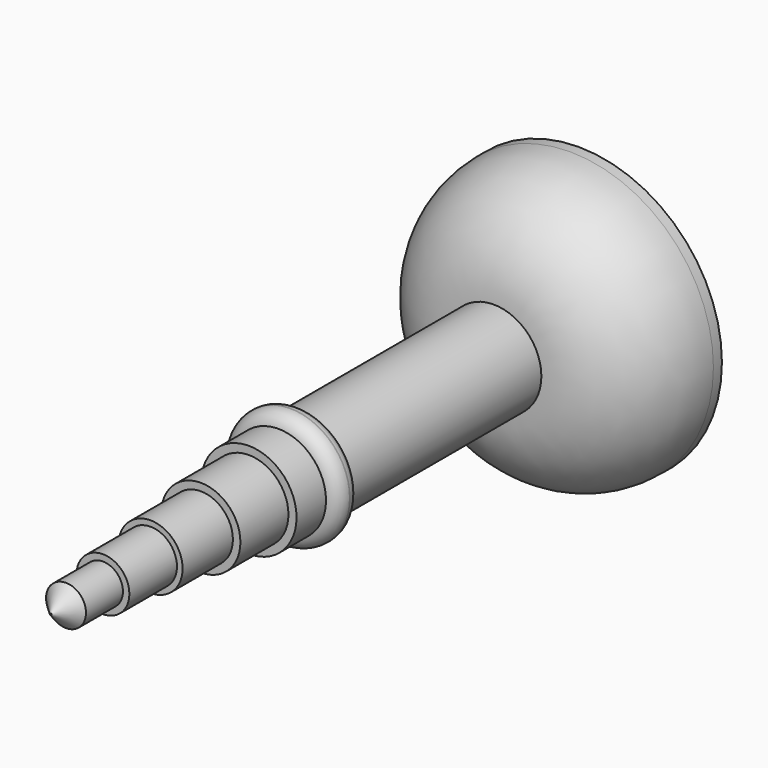
from build123d import *

# Parameters (mm, degrees)
F0_R      = 34.2582763281
F1_DEPTH  = 25.4
F2_R      = 22.86
F3_DEPTH  = 57.9221248627
F4_R      = 14.2196111498
F4_R_2    = 11.3982763281
F5_DEPTH  = 6.4626615494
F7_R      = 2.794
F8_DEPTH  = 15.2733121067
F9_R      = 9.4619725581
F10_DEPTH = 14.3653638661
F11_R     = 7.6680324081
F12_DEPTH = 15.0388088077
F13_R     = 6.3210744691
F14_DEPTH = 14.2291132361
F15_R     = 4.7785740108
F16_DEPTH = 15.6039167196
F17_SIZE  = 4.572


# Not quite as in the source:
# - a fillet or chamfer that OpenCascade refuses, or shapes differently, is made with other operations: its cross-section is extruded or revolved along the edge and cut away or added


with BuildPart() as f1:
    # F0 (on Front) → F1 (new body)
    with BuildSketch(Plane.XZ):
        Circle(F0_R)
    extrude(amount=F1_DEPTH)

    # F2
    f2_edges = [f1.edges().sort_by_distance(p)[0] for p in [
        (-34.258276, -25.4, 0),
    ]]
    fillet(f2_edges, radius=F2_R)

    # F3 (add): a face of the model
    f3_faces = [f1.faces().sort_by_distance(p)[0] for p in [
        (0, -25.4, 0),
    ]]
    extrude(f3_faces, amount=F3_DEPTH)


with BuildPart() as f5:
    # F4 (on face) → F5 (new body)
    with BuildSketch(Plane.XZ.offset(83.3221248627)):
        Circle(F4_R)
        Circle(F4_R_2, mode=Mode.SUBTRACT)
    extrude(amount=F5_DEPTH)

    # F6: fillet of radius 3.556 on 1 edges, made by hand

    # F6_s1 → F6_t2 (revolve, cut)
    with BuildSketch(Plane.XY):
        with BuildLine():
            ThreePointArc((14.2196111498, -86.3055044351), (13.4256398765, -88.5452216746), (11.3982763281, -89.7847864121))
            Line((11.3982763281, -89.7847864121), (14.2196111498, -89.7847864121))
            Line((14.2196111498, -89.7847864121), (14.2196111498, -86.3055044351))
        make_face()
    revolve(axis=Axis((0, -89.7847864121, 0), (0, -1, 0)), mode=Mode.SUBTRACT)

    # F7
    f7_edges = [f5.edges().sort_by_distance(p)[0] for p in [
        (-14.219611, -83.322125, 0),
    ]]
    fillet(f7_edges, radius=F7_R)


with BuildPart() as f8:
    # F8 (new): a face of the model
    f8_faces = [f1.part.faces().sort_by_distance(p)[0] for p in [
        (0, -83.3221248627, 0),
    ]]
    extrude(f8_faces, amount=F8_DEPTH)

    # F9 (on face) → F10 (join)
    with BuildSketch(Plane.XZ.offset(98.5954369694)):
        Circle(F9_R)
    extrude(amount=F10_DEPTH)

    # F11 (on face) → F12 (join)
    with BuildSketch(Plane.XZ.offset(112.9608008355)):
        Circle(F11_R)
    extrude(amount=F12_DEPTH)

    # F13 (on face) → F14 (join)
    with BuildSketch(Plane.XZ.offset(127.9996096432)):
        Circle(F13_R)
    extrude(amount=F14_DEPTH)

    # F15 (on face) → F16 (join)
    with BuildSketch(Plane.XZ.offset(142.2287228793)):
        Circle(F15_R)
    extrude(amount=F16_DEPTH)

    # F17
    f17_edges = [f8.edges().sort_by_distance(p)[0] for p in [
        (-4.778574, -157.83264, 0),
    ]]
    chamfer(f17_edges, length=F17_SIZE)


solid = Compound([f1.part, f5.part, f8.part])
